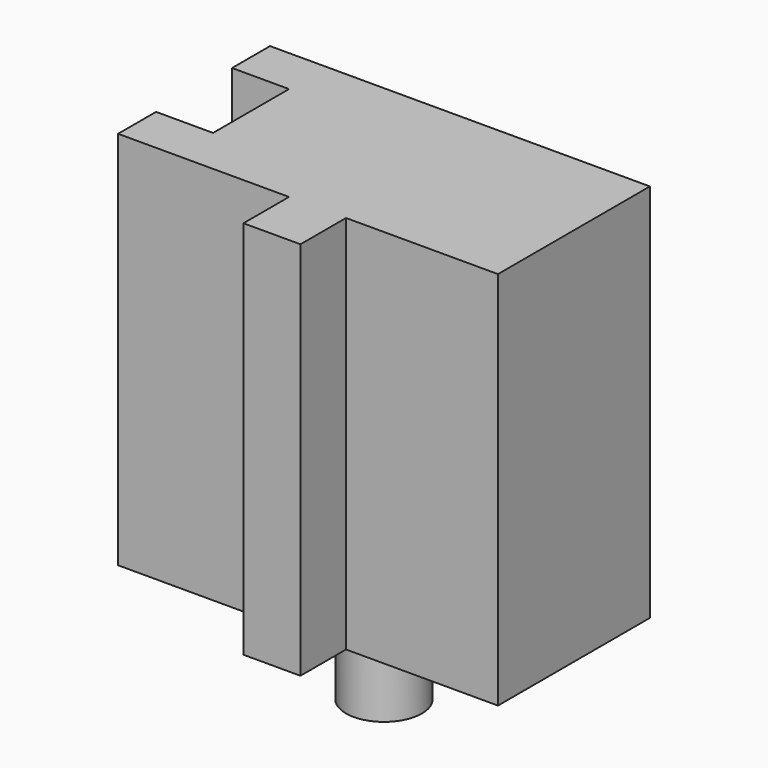
from build123d import *

# Parameters (mm, degrees)
F0_W     = 20
F0_H     = 10
F1_DEPTH = 20
F3_R     = 2
F4_DEPTH = 5
F5_DEPTH = 5
F2_W     = 3
F2_H     = 5
F6_DEPTH = 49
F2_H_2   = 3
F7_DEPTH = 20
F8_DEPTH = 20


# Not quite as in the source:
# - an extrude ends at something that could not be found from the text; its depth is read off the source's solid


with BuildPart() as f1:
    # F0 (on Top) → F1 (new body)
    with BuildSketch(Plane.XY):
        with Locations((10, 5)):
            Rectangle(F0_W, F0_H)
    extrude(amount=F1_DEPTH)

    # F3 (on face) → F4 (join)
    with BuildSketch(Plane(origin=(0, 0, 0), x_dir=(1, 0, 0), z_dir=(0, 0, -1))):
        with Locations((10, -5)):
            Circle(F3_R)
    extrude(amount=F4_DEPTH)

    # F3 (on face) → F5 (join)
    with BuildSketch(Plane(origin=(0, 0, 0), x_dir=(1, 0, 0), z_dir=(0, 0, -1))):
        with Locations((10, -5)):
            Circle(F3_R)
    extrude(amount=F5_DEPTH)

    # F2 (on face) → F6 (cut, through all)
    with BuildSketch(Plane.XY.offset(20)):
        with Locations((1.5, 5)):
            Rectangle(F2_W, F2_H)
    extrude(amount=-F6_DEPTH, mode=Mode.SUBTRACT)

    # F2 (on face) → F7 (join, through all)
    with BuildSketch(Plane.XY.offset(20)):
        with Locations((1.5, 5)):
            Rectangle(F2_W, F2_H)
        with Locations((10.5, -1.5)):
            Rectangle(F2_W, F2_H_2)
    extrude(amount=-F7_DEPTH)

    # F2 (on face) → F8 (cut, through all)
    with BuildSketch(Plane.XY.offset(20)):
        with Locations((1.5, 5)):
            Rectangle(F2_W, F2_H)
    extrude(amount=-F8_DEPTH, mode=Mode.SUBTRACT)


solid = f1.part
